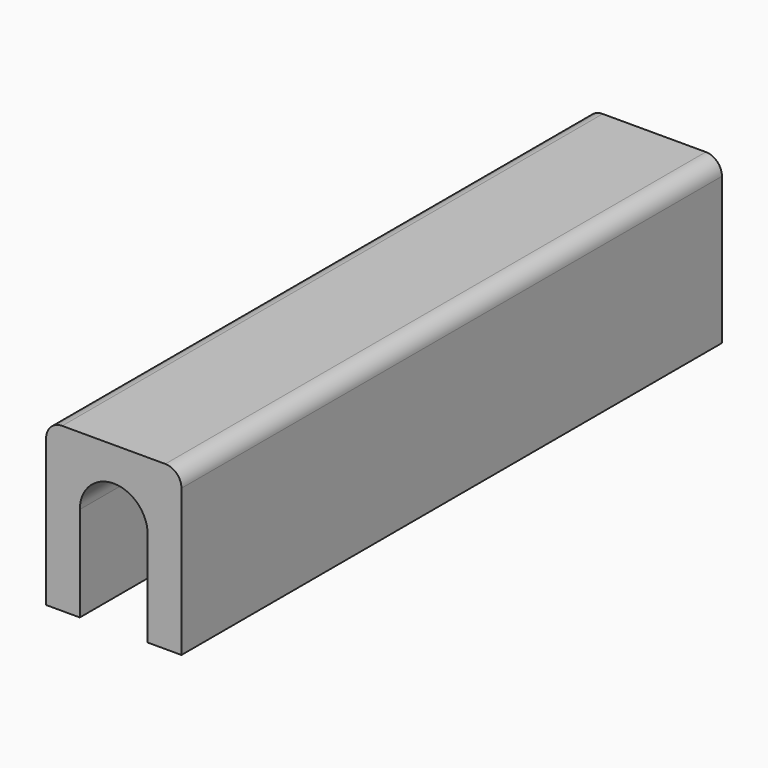
from build123d import *

# Parameters (mm, degrees)
F0_W     = 15.95
F0_H     = 19.2
F1_DEPTH = 79.6
F2_R     = 1.9
F3_W     = 8
F3_H     = 15.2
F4_DEPTH = 79.601
F5_R     = 3.99999


# Not quite as in the source:
# - a fillet or chamfer is up to 0.001 mm smaller than in the source, because OpenCascade refuses the exact size


with BuildPart() as f1:
    # F0 (on Front) → F1 (new body)
    with BuildSketch(Plane.XZ):
        with Locations((0, -1.6)):
            Rectangle(F0_W, F0_H)
    extrude(amount=-F1_DEPTH)

    # F2
    f2_edges = [f1.edges().sort_by_distance(p)[0] for p in [
        (7.975, 39.8, 8),
        (-7.975, 39.8, 8),
    ]]
    fillet(f2_edges, radius=F2_R)

    # F3 (on face) → F4 (cut, through all)
    with BuildSketch(Plane.XZ):
        with Locations((0, -3.6)):
            Rectangle(F3_W, F3_H)
    extrude(amount=-F4_DEPTH, mode=Mode.SUBTRACT)

    # F5 (radius 4 in the source; OpenCascade refuses exactly that, so slightly less here)
    f5_edges = [f1.edges().sort_by_distance(p)[0] for p in [
        (4, 39.8, 4),
        (-4, 39.8, 4),
    ]]
    fillet(f5_edges, radius=F5_R)


solid = f1.part
